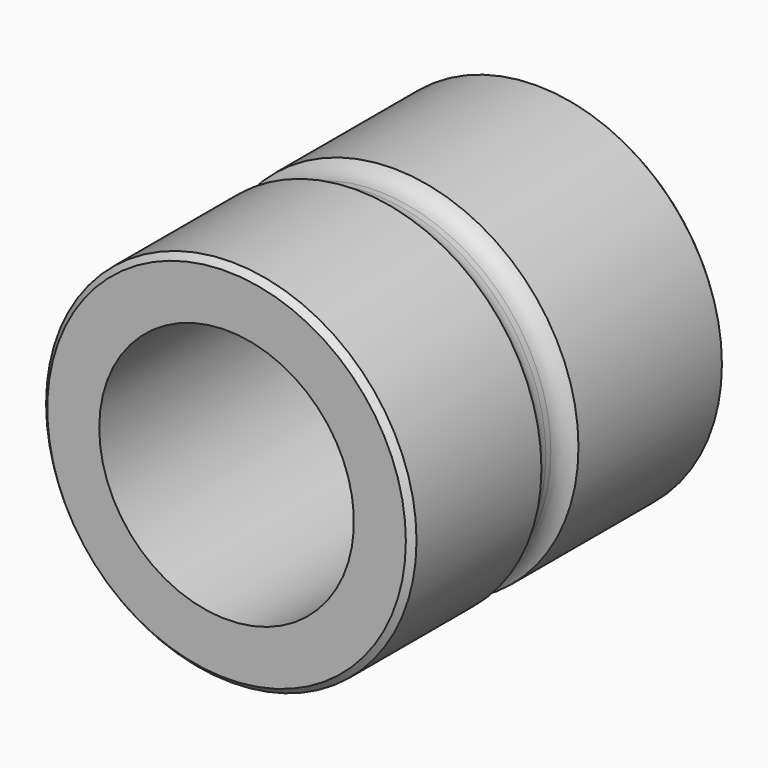
from build123d import *

# Parameters (mm, degrees)
F0_R      = 25.4
F0_R_2    = 17.4625
F1_DEPTH  = 25.4
F2_R      = 25.4
F2_R_2    = 23.8125
F3_DEPTH  = 3.175
F4_DEPTH  = 3.175
F5_R      = 25.4
F6_DEPTH  = 25.4
F8_SIZE   = 0.8128
F9_R      = 17.4625
F10_DEPTH = 53.976


# Not quite as in the source:
# - a fillet or chamfer that OpenCascade refuses, or shapes differently, is made with other operations: its cross-section is extruded or revolved along the edge and cut away or added


with BuildPart() as f1:
    # F0 (on Front) → F1 (new body)
    with BuildSketch(Plane.XZ):
        Circle(F0_R)
        Circle(F0_R_2, mode=Mode.SUBTRACT)
    extrude(amount=F1_DEPTH)

    # F2 (on face) → F3 (cut)
    with BuildSketch(Plane(origin=(0, 0, 0), x_dir=(-1, 0, 0), z_dir=(0, 1, 0))):
        Circle(F2_R)
        Circle(F2_R_2, mode=Mode.SUBTRACT)
    extrude(amount=-F3_DEPTH, mode=Mode.SUBTRACT)

    # F4 (add): a face of the model
    f4_faces = [f1.faces().sort_by_distance(p)[0] for p in [
        (23.1389807909, 0, 0),
    ]]
    extrude(f4_faces, amount=F4_DEPTH)

    # F5 (on face) → F6 (join)
    with BuildSketch(Plane(origin=(0, 3.175, 0), x_dir=(-1, 0, 0), z_dir=(0, 1, 0))):
        Circle(F5_R)
    extrude(amount=F6_DEPTH)

    # F7: fillet of radius 3.175 on 2 edges, made by hand

    # F7_s1 → F7_t2 (revolve)
    with BuildSketch(Plane.XY):
        with BuildLine():
            ThreePointArc((-23.8125, -0.425369343), (-24.237869343, -2.012869343), (-25.4, -3.175))
            Line((-25.4, -3.175), (-23.8125, -3.175))
            Line((-23.8125, -3.175), (-23.8125, -0.425369343))
        make_face()
    revolve(axis=Axis((0, -3.175, 0), (0, 1, 0)))

    # F7_s3 → F7_t4 (revolve)
    with BuildSketch(Plane.XY):
        with BuildLine():
            ThreePointArc((-25.4, 3.175), (-24.237869343, 2.012869343), (-23.8125, 0.425369343))
            Line((-23.8125, 0.425369343), (-23.8125, 3.175))
            Line((-23.8125, 3.175), (-25.4, 3.175))
        make_face()
    revolve(axis=Axis((0, 3.175, 0), (0, 1, 0)))

    # F8
    f8_edges = [f1.edges().sort_by_distance(p)[0] for p in [
        (-25.4, -25.4, 0),
        (25.4, 28.575, 0),
    ]]
    chamfer(f8_edges, length=F8_SIZE)

    # F9 (on face) → F10 (cut, through all)
    with BuildSketch(Plane(origin=(0, 28.575, 0), x_dir=(-1, 0, 0), z_dir=(0, 1, 0))):
        Circle(F9_R)
    extrude(amount=-F10_DEPTH, mode=Mode.SUBTRACT)


solid = f1.part
